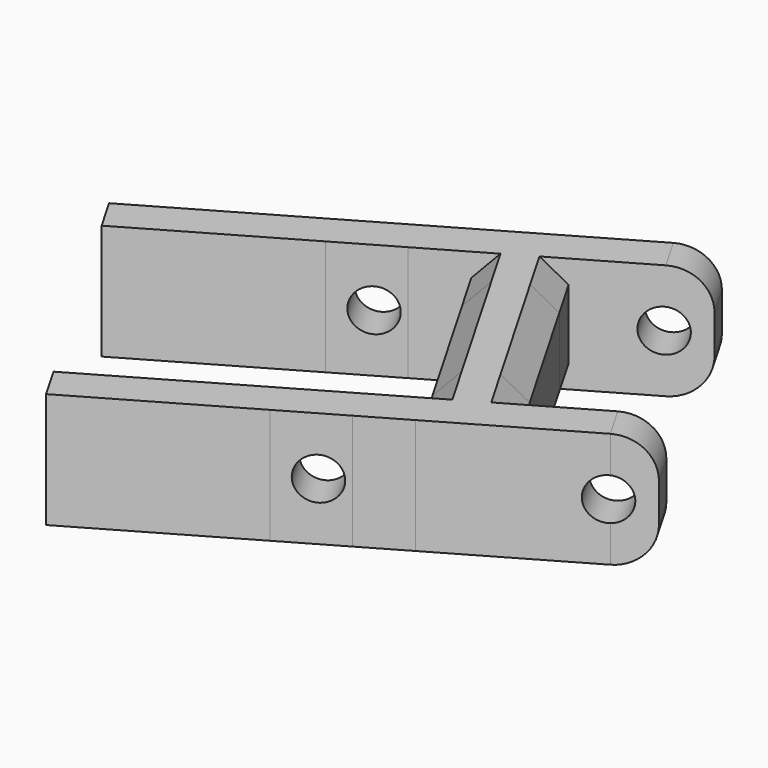
from build123d import *

# Parameters (mm, degrees)
F1_DEPTH = 15
F3_DEPTH = 60
F4_SIZE  = 3
F5_R     = 5


with BuildPart() as f1:
    # F0 (on Top) → F1 (new body)
    with BuildSketch(Plane.XY):
        Polygon((-84.375, 42.2187384345), (-78.75, 45.4663336987), (-61.4294919243, 55.4663336987), (-63.9294919243, 59.7964607176), (-72.5897459622, 54.7964607176), (-75.7147459622, 60.2091194913), (-84.375, 55.2091194913), (-81.25, 49.7964607176), (-86.875, 46.5488654534), align=None)
        Polygon((-61.4294919243, 55.4663336987), (-57.0993649054, 57.9663336987), (-59.5993649054, 62.2964607176), (-63.9294919243, 59.7964607176), align=None)
        Polygon((-91.7403810568, 37.9663336987), (-84.375, 42.2187384345), (-86.875, 46.5488654534), (-94.2403810568, 42.2964607176), align=None)
        Polygon((-84.375, 55.2091194913), (-75.7147459622, 60.2091194913), (-85.7147459622, 77.5296275669), (-87.793790014, 76.329290924), (-94.375, 72.5296275669), align=None)
        Polygon((-111.6589653438, 26.4663336987), (-91.7403810568, 37.9663336987), (-94.2403810568, 42.2964607176), (-114.1589653438, 30.7964607176), align=None)
        Polygon((-87.793790014, 76.329290924), (-85.7147459622, 77.5296275669), (-88.8397459622, 82.9422863406), (-75.8493649054, 90.4422863406), (-78.3493115936, 94.7723526968), (-100, 82.2724133595), (-105.625, 79.0248180953), (-103.125, 74.6946910764), (-97.5, 77.9422863406), (-94.375, 72.5296275669), align=None)
        Polygon((-110.4903810568, 70.4422863406), (-103.125, 74.6946910764), (-105.625, 79.0248180953), (-112.9903810568, 74.7724133595), align=None)
        Polygon((-130.4089653438, 58.9422863406), (-110.4903810568, 70.4422863406), (-112.9903810568, 74.7724133595), (-132.9089653438, 63.2724133595), align=None)
    extrude(amount=F1_DEPTH)

    # F2 (on face) → F3 (cut)
    with BuildSketch(Plane(origin=(-39.375, 68.199500548, 0), x_dir=(0.8660254038, 0.5, 0), z_dir=(0.5, -0.8660254038, 0))):
        with BuildLine():
            ThreePointArc((-52.7163336987, 7.5), (-55.4663336987, 10.25), (-58.2163336987, 7.5))
            Line((-58.2163336987, 7.5), (-55.4663336987, 7.5))
            Line((-55.4663336987, 7.5), (-52.7163336987, 7.5))
        make_face()
        with BuildLine():
            Line((-55.4663336987, 7.5), (-58.2163336987, 7.5))
            ThreePointArc((-58.2163336987, 7.5), (-55.4663336987, 4.75), (-52.7163336987, 7.5))
            Line((-52.7163336987, 7.5), (-55.4663336987, 7.5))
        make_face()
        with BuildLine():
            ThreePointArc((-22.8953336987, 7.5), (-25.6453336987, 10.25), (-28.3953336987, 7.5))
            ThreePointArc((-28.3953336987, 7.5), (-25.6453336987, 4.75), (-22.8953336987, 7.5))
        make_face()
    extrude(amount=-F3_DEPTH, mode=Mode.SUBTRACT)

    # F4
    f4_edges = [f1.edges().sort_by_distance(p)[0] for p in [
        (-89.375, 63.869374, 15),
        (-80.714746, 68.869374, 15),
        (-89.375, 63.869374, 0),
        (-80.714746, 68.869374, 0),
    ]]
    chamfer(f4_edges, length=F4_SIZE)

    # F5
    f5_edges = [f1.edges().sort_by_distance(p)[0] for p in [
        (-58.349365, 60.131397, 15),
        (-58.349365, 60.131397, 0),
        (-77.099338, 92.60732, 15),
        (-77.099338, 92.60732, 0),
    ]]
    fillet(f5_edges, radius=F5_R)


solid = f1.part
